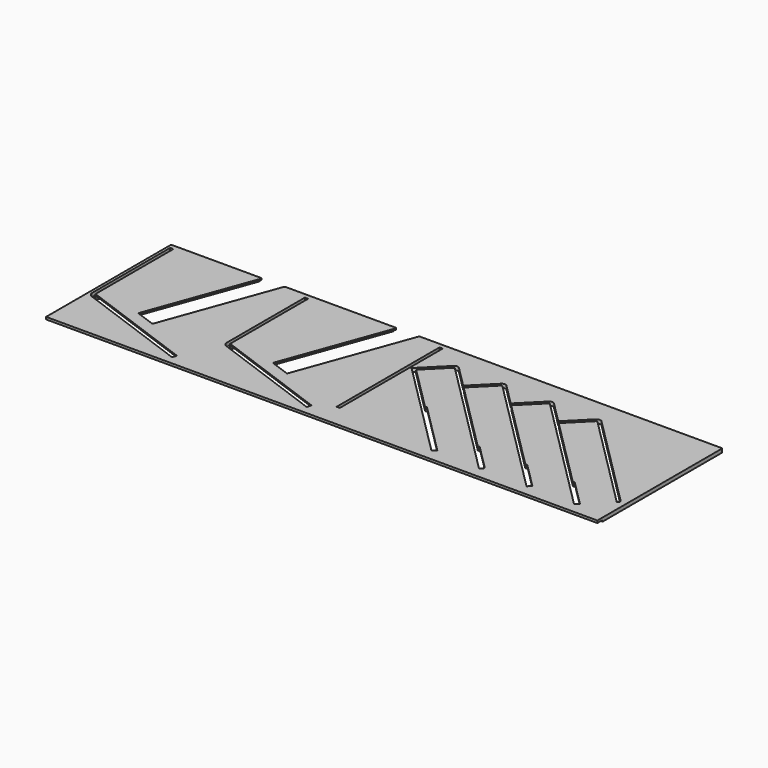
from build123d import *

# Parameters (mm, degrees)
F0_W     = 3.5
F0_H     = 140
F1_DEPTH = 4
F3_DEPTH = 2.5
F2_W     = 599.6014092535
F2_H     = 7
F4_DEPTH = 1.5


# Not quite as in the source:
# - a feature names something its author has since deleted; it is built from what else it names


with BuildPart() as f1:
    # F0 (on Top) → F1 (new body)
    with BuildSketch(Plane.XY):
        with BuildLine():
            Line((-300.1670946785, -88.5), (299.4343145751, -88.5))
            Line((299.4343145751, -88.5), (299.4343145751, 80.5))
            ThreePointArc((299.4343145751, 80.5), (299.1414213562, 81.2071067812), (298.4343145751, 81.5))
            Line((298.4343145751, 81.5), (-29.5426009536, 81.5))
            ThreePointArc((-29.5426009536, 81.5), (-30.1161773899, 81.3191520443), (-30.4822935744, 80.8420201433))
            Line((-30.4822935744, 80.8420201433), (-32.577653202, 75.0850668809))
            Line((-32.577653202, 75.0850668809), (-74.89635139, -41.1846008115))
            ThreePointArc((-74.89635139, -41.1846008115), (-75.413425749, -41.7488884552), (-76.1780641541, -41.7822732889))
            Line((-76.1780641541, -41.7822732889), (-95.9102779047, -34.6003348275))
            ThreePointArc((-95.9102779047, -34.6003348275), (-96.4745655484, -34.0832604685), (-96.5079503821, -33.3186220634))
            Line((-96.5079503821, -33.3186220634), (-55.2058449976, 80.1579798567))
            ThreePointArc((-55.2058449976, 80.1579798567), (-55.3263855741, 81.0735764364), (-56.1455376183, 81.5))
            Line((-56.1455376183, 81.5), (-175.9202302026, 81.5))
            ThreePointArc((-175.9202302026, 81.5), (-176.4938066389, 81.3191520443), (-176.8599228233, 80.8420201433))
            Line((-176.8599228233, 80.8420201433), (-178.9462015538, 75.1100164406))
            Line((-178.9462015538, 75.1100164406), (-221.2882952976, -41.2239300127))
            ThreePointArc((-221.2882952976, -41.2239300127), (-221.8053696566, -41.7882176564), (-222.5700080617, -41.8216024902))
            Line((-222.5700080617, -41.8216024902), (-242.3022218123, -34.6396640288))
            ThreePointArc((-242.3022218123, -34.6396640288), (-242.866509456, -34.1225896697), (-242.8998942897, -33.3579512647))
            Line((-242.8998942897, -33.3579512647), (-201.5834742465, 80.1579798567))
            ThreePointArc((-201.5834742465, 80.1579798567), (-201.704014823, 81.0735764364), (-202.5231668673, 81.5))
            Line((-202.5231668673, 81.5), (-299.1670946785, 81.5))
            ThreePointArc((-299.1670946785, 81.5), (-299.8742014597, 81.2071067812), (-300.1670946785, 80.5))
            Line((-300.1670946785, 80.5), (-300.1670946785, -88.5))
        make_face()
        with BuildLine():
            ThreePointArc((182.4185499288, 56.2932249718), (185.2469770535, 57.4647978471), (188.0754041783, 56.2932249718))
            Line((188.0754041783, 56.2932249718), (293.4343145751, -49.0656854249))
            Line((293.4343145751, -49.0656854249), (290.9594408409, -51.5405591591))
            Line((290.9594408409, -51.5405591591), (185.9540838347, 53.4647978471))
            ThreePointArc((185.9540838347, 53.4647978471), (185.2469770535, 53.7576910659), (184.5398702723, 53.4647978471))
            Line((184.5398702723, 53.4647978471), (162.6195600555, 31.5444876303))
            ThreePointArc((162.6195600555, 31.5444876303), (162.3266668367, 30.8373808491), (162.6195600555, 30.1302740679))
            Line((162.6195600555, 30.1302740679), (238.6335390331, -45.8837049096))
            ThreePointArc((238.6335390331, -45.8837049096), (239.3406458143, -46.1765981284), (240.0477525955, -45.8837049096))
            Line((240.0477525955, -45.8837049096), (240.4013059861, -45.530151519))
            Line((240.4013059861, -45.530151519), (268.6855772335, -73.8144227665))
            Line((268.6855772335, -73.8144227665), (267.6249170617, -74.8750829383))
            Line((267.6249170617, -74.8750829383), (265.1500433276, -77.3499566724))
            Line((265.1500433276, -77.3499566724), (156.962705806, 30.8373808491))
            Line((156.962705806, 30.8373808491), (133.9817354175, 53.8183512377))
            ThreePointArc((133.9817354175, 53.8183512377), (133.2746286363, 54.1112444565), (132.5675218551, 53.8183512377))
            Line((132.5675218551, 53.8183512377), (110.6472116383, 31.8980410209))
            ThreePointArc((110.6472116383, 31.8980410209), (110.3543184195, 31.1909342397), (110.6472116383, 30.4838274585))
            Line((110.6472116383, 30.4838274585), (186.6611906159, -45.530151519))
            ThreePointArc((186.6611906159, -45.530151519), (187.3682973971, -45.8230447378), (188.0754041783, -45.530151519))
            Line((188.0754041783, -45.530151519), (188.4289575688, -45.1765981284))
            Line((188.4289575688, -45.1765981284), (216.7132288163, -73.4608693759))
            Line((216.7132288163, -73.4608693759), (215.6525686445, -74.5215295477))
            Line((215.6525686445, -74.5215295477), (213.1776949104, -76.9964032818))
            Line((213.1776949104, -76.9964032818), (104.9903573888, 31.1909342397))
            Line((104.9903573888, 31.1909342397), (82.0093870003, 54.1719046283))
            ThreePointArc((82.0093870003, 54.1719046283), (81.3022802191, 54.4647978471), (80.5951734379, 54.1719046283))
            Line((80.5951734379, 54.1719046283), (58.6748632211, 32.2515944115))
            ThreePointArc((58.6748632211, 32.2515944115), (58.3819700023, 31.5444876303), (58.6748632211, 30.8373808491))
            Line((58.6748632211, 30.8373808491), (134.6888421987, -45.1765981284))
            ThreePointArc((134.6888421987, -45.1765981284), (135.3959489799, -45.4694913472), (136.103055761, -45.1765981284))
            Line((136.103055761, -45.1765981284), (136.4566091516, -44.8230447378))
            Line((136.4566091516, -44.8230447378), (164.7408803991, -73.1073159853))
            Line((164.7408803991, -73.1073159853), (163.6802202273, -74.1679761571))
            Line((163.6802202273, -74.1679761571), (161.2053464932, -76.6428498912))
            Line((161.2053464932, -76.6428498912), (53.0180089716, 31.5444876303))
            Line((53.0180089716, 31.5444876303), (30.0370385831, 54.5254580189))
            ThreePointArc((30.0370385831, 54.5254580189), (29.3299318019, 54.8183512377), (28.6228250207, 54.5254580189))
            Line((28.6228250207, 54.5254580189), (6.7025148039, 32.6051478021))
            ThreePointArc((6.7025148039, 32.6051478021), (6.4096215851, 31.8980410209), (6.7025148039, 31.1909342397))
            Line((6.7025148039, 31.1909342397), (54.432222534, -16.5387734904))
            ThreePointArc((54.432222534, -16.5387734904), (55.1393293152, -16.8316667092), (55.8464360964, -16.5387734904))
            Line((55.8464360964, -16.5387734904), (56.199989487, -16.1852200998))
            Line((56.199989487, -16.1852200998), (112.7685319819, -72.7537625947))
            Line((112.7685319819, -72.7537625947), (111.7078718101, -73.8144227665))
            Line((111.7078718101, -73.8144227665), (109.232998076, -76.2892965006))
            Line((109.232998076, -76.2892965006), (1.0456605544, 31.8980410209))
            Line((1.0456605544, 31.8980410209), (26.5015046771, 57.3538851436))
            ThreePointArc((26.5015046771, 57.3538851436), (29.3299318019, 58.5254580189), (32.1583589266, 57.3538851436))
            Line((32.1583589266, 57.3538851436), (55.4928827058, 34.0193613645))
            Line((55.4928827058, 34.0193613645), (78.4738530943, 57.000331753))
            ThreePointArc((78.4738530943, 57.000331753), (81.3022802191, 58.1719046283), (84.1307073438, 57.000331753))
            Line((84.1307073438, 57.000331753), (107.465231123, 33.6658079739))
            Line((107.465231123, 33.6658079739), (130.4462015116, 56.6467783624))
            ThreePointArc((130.4462015116, 56.6467783624), (133.2746286363, 57.8183512377), (136.103055761, 56.6467783624))
            Line((136.103055761, 56.6467783624), (159.4375795402, 33.3122545833))
            Line((159.4375795402, 33.3122545833), (182.4185499288, 56.2932249718))
        make_face(mode=Mode.SUBTRACT)
        with BuildLine():
            Line((-297.1670946785, -29.2987547707), (-297.1670946785, 76.5))
            Line((-297.1670946785, 76.5), (-293.6670946785, 76.5))
            Line((-293.6670946785, 76.5), (-293.6670946785, -28.9486510016))
            ThreePointArc((-293.6670946785, -28.9486510016), (-293.1245508114, -30.6693803107), (-291.6931551085, -31.767728864))
            Line((-291.6931551085, -31.767728864), (-291.1801248935, -30.3581899328))
            Line((-291.1801248935, -30.3581899328), (-247.9542643373, -46.0911165258))
            Line((-247.9542643373, -46.0911165258), (-216.0047152306, -57.7198013989))
            Line((-216.0047152306, -57.7198013989), (-169.1115203708, -74.7875285175))
            Line((-169.1115203708, -74.7875285175), (-169.1115203708, -76.3837951762))
            Line((-169.1115203708, -76.3837951762), (-170.3085908724, -79.672719349))
            Line((-170.3085908724, -79.672719349), (-293.2192155384, -34.9369104955))
            ThreePointArc((-293.2192155384, -34.9369104955), (-296.0820069442, -32.7402133888), (-297.1670946785, -29.2987547707))
        make_face(mode=Mode.SUBTRACT)
        with BuildLine():
            Line((-150.6670946785, -29.2987547707), (-150.6670946785, 76.5))
            Line((-150.6670946785, 76.5), (-147.1670946785, 76.5))
            Line((-147.1670946785, 76.5), (-147.1670946785, -28.9486510016))
            ThreePointArc((-147.1670946785, -28.9486510016), (-146.6245508114, -30.6693803107), (-145.1931551085, -31.767728864))
            Line((-145.1931551085, -31.767728864), (-144.6801248935, -30.3581899328))
            Line((-144.6801248935, -30.3581899328), (-101.4542643373, -46.0911165258))
            Line((-101.4542643373, -46.0911165258), (-69.5047152306, -57.7198013989))
            Line((-69.5047152306, -57.7198013989), (-22.6115203708, -74.7875285175))
            Line((-22.6115203708, -74.7875285175), (-22.6115203708, -76.3837951762))
            Line((-22.6115203708, -76.3837951762), (-23.8085908724, -79.672719349))
            Line((-23.8085908724, -79.672719349), (-146.7192155384, -34.9369104955))
            ThreePointArc((-146.7192155384, -34.9369104955), (-149.5820069442, -32.7402133888), (-150.6670946785, -29.2987547707))
        make_face(mode=Mode.SUBTRACT)
        with Locations((-2.4170946785, 6.5)):
            Rectangle(F0_W, F0_H, mode=Mode.SUBTRACT)
    extrude(amount=F1_DEPTH)

    # F2 (on face) → F3 (cut)
    with BuildSketch(Plane(origin=(0, 0, 0), x_dir=(1, 0, 0), z_dir=(0, 0, -1))):
        Polygon((275.7566450454, 66.7433549546), (268.6855772335, 73.8144227665), (240.4013059861, 45.530151519), (247.4723737979, 38.4590837072), align=None)
        Polygon((216.7132288163, 73.4608693759), (188.4289575688, 45.1765981284), (195.5000253807, 38.1055303166), (223.7842966282, 66.389801564), align=None)
        Polygon((164.7408803991, 73.1073159853), (136.4566091516, 44.8230447378), (143.5276769635, 37.751976926), (171.811948211, 66.0362481734), align=None)
        Polygon((119.8395997938, 65.6826947828), (112.7685319819, 72.7537625947), (56.199989487, 16.1852200998), (63.2710572988, 9.1141522879), align=None)
        with BuildLine():
            Line((-26.1847247522, -84.1663356758), (-27.1494019864, -81.5))
            Line((-27.1494019864, -81.5), (-29.5426009536, -81.5))
            ThreePointArc((-29.5426009536, -81.5), (-30.1161773899, -81.3191520443), (-30.4822935744, -80.8420201433))
            Line((-30.4822935744, -80.8420201433), (-74.89635139, 41.1846008115))
            ThreePointArc((-74.89635139, 41.1846008115), (-75.413425749, 41.7488884552), (-76.1780641541, 41.7822732889))
            Line((-76.1780641541, 41.7822732889), (-95.9102779047, 34.6003348275))
            ThreePointArc((-95.9102779047, 34.6003348275), (-96.4745655484, 34.0832604685), (-96.5079503821, 33.3186220634))
            Line((-96.5079503821, 33.3186220634), (-55.2058449976, -80.1579798567))
            ThreePointArc((-55.2058449976, -80.1579798567), (-55.3263855741, -81.0735764364), (-56.1455376183, -81.5))
            Line((-56.1455376183, -81.5), (-57.8035051482, -81.5))
            Line((-57.8035051482, -81.5), (-56.1411243122, -86.0673538194))
            Line((-56.1411243122, -86.0673538194), (-53.1341079256, -84.9728893607))
            Line((-53.1341079256, -84.9728893607), (-96.2260425959, 33.4212281064))
            Line((-96.2260425959, 33.4212281064), (-75.1769278903, 41.0824793169))
            Line((-75.1769278903, 41.0824793169), (-29.193835551, -85.2550285621))
            Line((-29.193835551, -85.2550285621), (-26.1847247522, -84.1663356758))
        make_face()
        with BuildLine():
            Line((-29.5426009536, -81.5), (-27.1494019864, -81.5))
            Line((-27.1494019864, -81.5), (-73.0435823042, 45.3499825234))
            Line((-73.0435823042, 45.3499825234), (-18.4155032039, 65.2329772711))
            Line((-18.4155032039, 65.2329772711), (-21.9858379993, 75.3345116245))
            Line((-21.9858379993, 75.3345116245), (-22.6115203708, 75.1067818652))
            Line((-22.6115203708, 75.1067818652), (-22.6115203708, 74.7875285175))
            Line((-22.6115203708, 74.7875285175), (-144.6801248935, 30.3581899328))
            Line((-144.6801248935, 30.3581899328), (-144.7827309416, 30.6400977331))
            Line((-144.7827309416, 30.6400977331), (-144.7829091425, 30.6400328733))
            Line((-144.7829091425, 30.6400328733), (-141.1916976375, 20.7732603551))
            Line((-141.1916976375, 20.7732603551), (-100.4280628419, 35.6100100293))
            Line((-100.4280628419, 35.6100100293), (-57.8035051482, -81.5))
            Line((-57.8035051482, -81.5), (-56.1455376183, -81.5))
            ThreePointArc((-56.1455376183, -81.5), (-55.3263855741, -81.0735764364), (-55.2058449976, -80.1579798567))
            Line((-55.2058449976, -80.1579798567), (-96.5079503821, 33.3186220634))
            ThreePointArc((-96.5079503821, 33.3186220634), (-96.4745655484, 34.0832604685), (-95.9102779047, 34.6003348275))
            Line((-95.9102779047, 34.6003348275), (-76.1780641541, 41.7822732889))
            ThreePointArc((-76.1780641541, 41.7822732889), (-75.413425749, 41.7488884552), (-74.89635139, 41.1846008115))
            Line((-74.89635139, 41.1846008115), (-30.4822935744, -80.8420201433))
            ThreePointArc((-30.4822935744, -80.8420201433), (-30.1161773899, -81.3191520443), (-29.5426009536, -81.5))
        make_face()
        with BuildLine():
            Line((-246.8200068386, 35.6493392141), (-204.1811344008, -81.5))
            Line((-204.1811344008, -81.5), (-202.5231668673, -81.5))
            ThreePointArc((-202.5231668673, -81.5), (-201.704014823, -81.0735764364), (-201.5834742465, -80.1579798567))
            Line((-201.5834742465, -80.1579798567), (-242.8998942897, 33.3579512647))
            ThreePointArc((-242.8998942897, 33.3579512647), (-242.866509456, 34.1225896697), (-242.3022218123, 34.6396640288))
            Line((-242.3022218123, 34.6396640288), (-222.5700080617, 41.8216024902))
            ThreePointArc((-222.5700080617, 41.8216024902), (-221.8053696566, 41.7882176564), (-221.2882952976, 41.2239300127))
            Line((-221.2882952976, 41.2239300127), (-176.8599228233, -80.8420201433))
            ThreePointArc((-176.8599228233, -80.8420201433), (-176.4938066389, -81.3191520443), (-175.9202302026, -81.5))
            Line((-175.9202302026, -81.5), (-173.5328145535, -81.5))
            Line((-173.5328145535, -81.5), (-219.7344579026, 45.4379718434))
            Line((-219.7344579026, 45.4379718434), (-165.206104517, 65.2846693993))
            Line((-165.206104517, 65.2846693993), (-168.2128599899, 75.4338674786))
            Line((-168.2128599899, 75.4338674786), (-169.1115203708, 75.1067818492))
            Line((-169.1115203708, 75.1067818492), (-169.1115203708, 74.7875285175))
            Line((-169.1115203708, 74.7875285175), (-291.1801248935, 30.3581899328))
            Line((-291.1801248935, 30.3581899328), (-287.6915194316, 20.7733252008))
            Line((-287.6915194316, 20.7733252008), (-246.8200068386, 35.6493392141))
        make_face()
    extrude(amount=-F3_DEPTH, mode=Mode.SUBTRACT)

    # F2 (on face) → F4 (cut)
    with BuildSketch(Plane(origin=(0, 0, 0), x_dir=(1, 0, 0), z_dir=(0, 0, -1))):
        with Locations((-0.3663900517, 85)):
            Rectangle(F2_W, F2_H)
    extrude(amount=-F4_DEPTH, mode=Mode.SUBTRACT)


solid = f1.part
